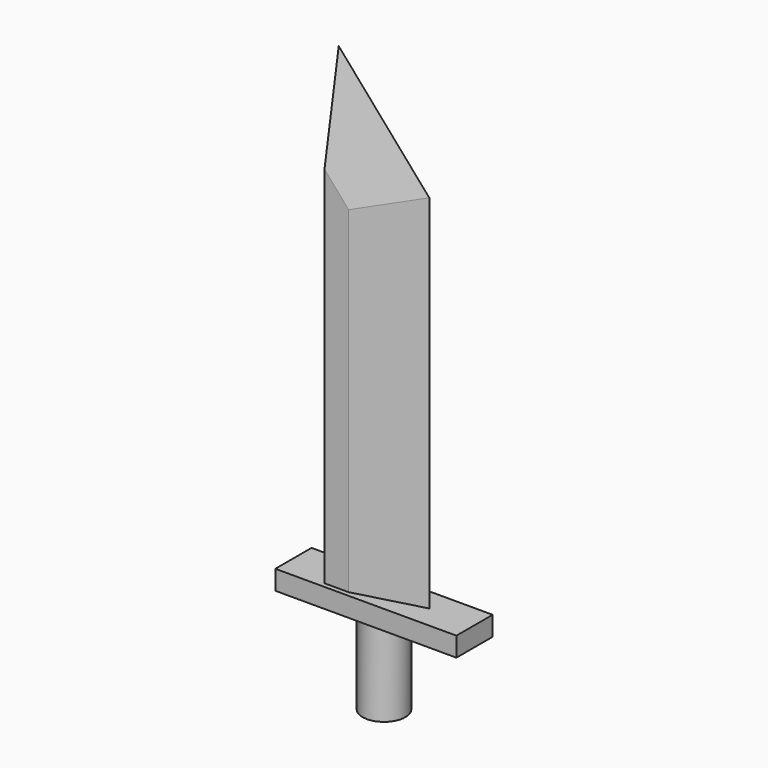
from build123d import *

# Parameters (mm, degrees)
F0_R       = 16.5
F1_DEPTH   = 80
F2_W       = 140
F2_H       = 35
F2_R       = 16.5
F3_DEPTH   = 15
F4_W       = 70
F4_H       = 27.5
F5_DEPTH   = 360
F7_DEPTH   = 50
F8_SIZE2   = 13.75
F8_SIZE    = 51.3156986041
F8_2_SIZE2 = 13.74999
F8_2_SIZE  = 51.315689


# Not quite as in the source:
# - a fillet or chamfer is up to 0.001 mm smaller than in the source, because OpenCascade refuses the exact size


with BuildPart() as f1:
    # F0 (on Top) → F1 (new body)
    with BuildSketch(Plane.XY):
        Circle(F0_R)
    extrude(amount=-F1_DEPTH)

    # F2 (on face) → F3 (join)
    with BuildSketch(Plane.XY):
        Rectangle(F2_W, F2_H)
        Circle(F2_R, mode=Mode.SUBTRACT)
    extrude(amount=-F3_DEPTH)

    # F4 (on face) → F5 (join)
    with BuildSketch(Plane.XY):
        Rectangle(F4_W, F4_H)
    extrude(amount=F5_DEPTH)

    # F6 (on face) → F7 (cut)
    with BuildSketch(Plane.XZ.offset(13.75)):
        Polygon((35, 360), (-35, 360), (35, 279.5273661613), align=None)
    extrude(amount=-F7_DEPTH, mode=Mode.SUBTRACT)

    # F8
    f8_edges = [f1.edges().sort_by_distance(p)[0] for p in [
        (35, 13.75, 139.763683),
        (0, 13.75, 319.763683),
    ]]
    f8_side = f1.faces().sort_by_distance((-1.468033, 13.75, 160.725674))[0]
    chamfer(f8_edges, length=F8_SIZE, length2=F8_SIZE2, reference=f8_side)

    # F8#2 (size 51.3156986041 and 13.75 in the source; OpenCascade refuses exactly that, so slightly less here)
    f8_2_edges = [f1.edges().sort_by_distance(p)[0] for p in [
        (35, -13.75, 139.763683),
        (0, -13.75, 319.763683),
    ]]
    f8_2_side = f1.faces().sort_by_distance((-1.468033, -13.75, 160.725674))[0]
    chamfer(f8_2_edges, length=F8_2_SIZE, length2=F8_2_SIZE2, reference=f8_2_side)


solid = f1.part
